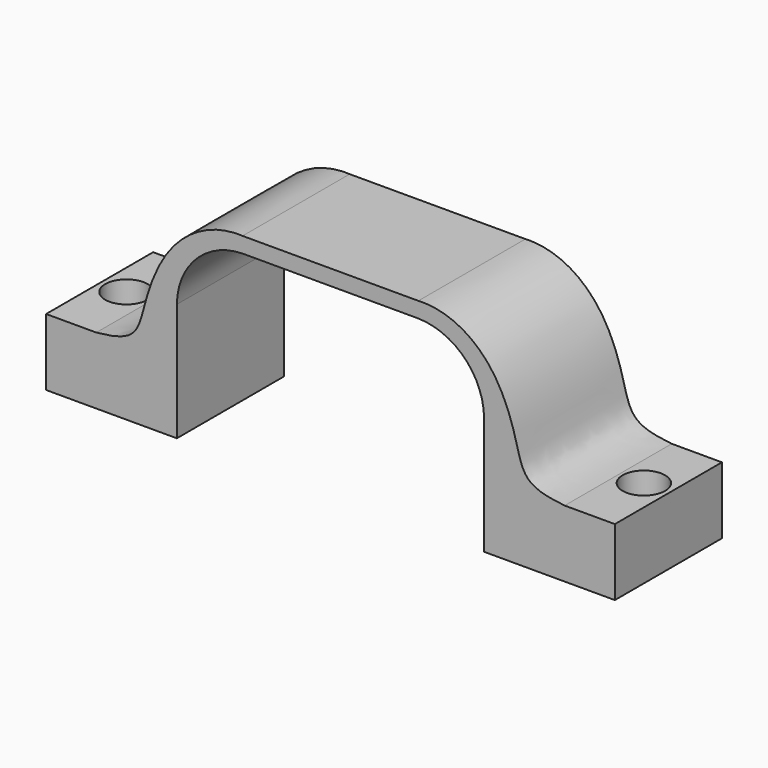
from build123d import *

# Parameters (mm, degrees)
F3_DEPTH = 20
F5_D     = 6.35
F6_D     = 6.35


with BuildPart() as f3:
    # F2 (on Front) → F3 (new body)
    with BuildSketch(Plane.XZ):
        with BuildLine():
            Line((0, 29.8221680522), (-13.1319385877, 29.8221680522))
            add(Edge.make_bspline(
                [(-35, 10), (-31.0387470191, 10.3774955025), (-28.7332573155, 11.8333441201), (-27.7320793476, 16.5781182185), (-24.7421079623, 25.5876719553), (-17.7754473796, 30.0339317742), (-13.1319385877, 29.8221680522)],
                knots=[0, 0, 0, 0, 0.2304435878, 0.4134879343, 0.6870551645, 1, 1, 1, 1], degree=3))
            Line((-35, 10), (-42.5, 10))
            Line((-42.5, 10), (-42.5, 0))
            Line((-42.5, 0), (-22.9563365987, 0))
            Line((-22.9563365987, 0), (-22.9563365987, 10))
            Line((-22.9563365987, 10), (-22.9563365987, 17.6236335862))
            ThreePointArc((-22.9563365987, 17.6236335862), (-20.0327244278, 24.5669984184), (-13.093320632, 27.5))
            Line((-13.093320632, 27.5), (0, 27.5))
            Line((0, 27.5), (13.093320632, 27.5))
            ThreePointArc((13.093320632, 27.5), (20.0327244278, 24.5669984184), (22.9563365987, 17.6236335862))
            Line((22.9563365987, 17.6236335862), (22.9563365987, 10))
            Line((22.9563365987, 10), (22.9563365987, 0))
            Line((22.9563365987, 0), (42.5, 0))
            Line((42.5, 0), (42.5, 10))
            Line((42.5, 10), (35, 10))
            add(Edge.make_bspline(
                [(35, 10), (31.0387470191, 10.3774955025), (28.7332573155, 11.8333441201), (27.7320793476, 16.5781182185), (24.7421079623, 25.5876719553), (17.7754473796, 30.0339317742), (13.1319385877, 29.8221680522)],
                knots=[0, 0, 0, 0, 0.2304435878, 0.4134879343, 0.6870551645, 1, 1, 1, 1], degree=3))
            Line((13.1319385877, 29.8221680522), (0, 29.8221680522))
        make_face()
    extrude(amount=F3_DEPTH)

    # F5 (through all)
    with Locations(Plane(origin=(0, 0, 0), x_dir=(1, 0, 0), z_dir=(0, 0, -1))):
        with Locations((-38.6619865894, 9.7850039601)):
            Hole(F5_D / 2)

    # F6 (through all)
    with Locations(Plane(origin=(0, 0, 0), x_dir=(1, 0, 0), z_dir=(0, 0, -1))):
        with Locations((38.6619865894, 9.7850039601)):
            Hole(F6_D / 2)


solid = f3.part
